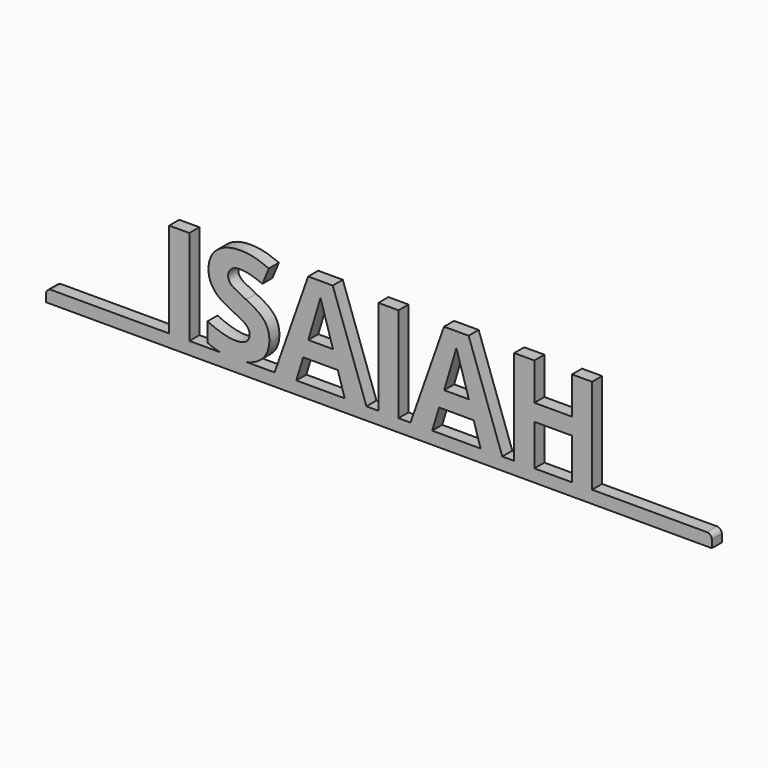
from build123d import *

# Parameters (mm, degrees)
F0_W         = 673.1
F0_H         = 12.7
F1_DEPTH     = 12.7
F2_TEXT_SIZE = 134.5296568962
F3_DEPTH     = 12.7
F4_R         = 5.08


# Not quite as in the source:
# - Text() gives the source's letters only with a copy of the font that has no kerning and outlines rounded to 1/6400 em; it was checked with that copy


with BuildPart() as f1:
    # F0 (on Front) → F1 (new body)
    with BuildSketch(Plane.XZ):
        with Locations((0, -25.1498585314)):
            Rectangle(F0_W, F0_H)
    extrude(amount=F1_DEPTH)

    # F2 (on face) → F3 (join)
    with BuildSketch(Plane.XZ.offset(12.7)):
        with Locations((-224.1705509327, -18.7998585314)):
            Text('ISAIAH', F2_TEXT_SIZE, font='Open Sans', font_style=FontStyle.BOLD, text_align=(TextAlign.LEFT, TextAlign.BOTTOM))
    extrude(amount=-F3_DEPTH)

    # F4
    f4_edges = [f1.edges().sort_by_distance(p)[0] for p in [
        (336.55, -6.35, -18.799859),
        (-336.55, -6.35, -18.799859),
    ]]
    fillet(f4_edges, radius=F4_R)


solid = f1.part
